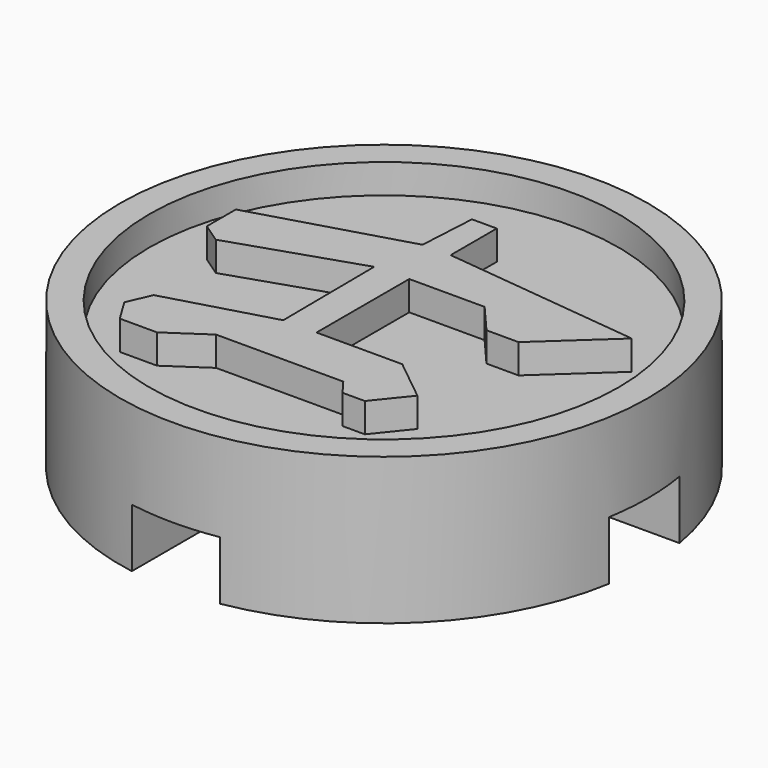
from build123d import *

# Parameters (mm, degrees)
F0_R     = 9
F1_DEPTH = 4
F3_W     = 3
F3_H     = 3
F4_DEPTH = 2
F2_R     = 9
F2_R_2   = 8
F5_DEPTH = 1


with BuildPart() as f1:
    # F0 (on Top) → F1 (new body)
    with BuildSketch(Plane.XY):
        with Locations((-31.3306450844, 19.7580661625)):
            Circle(F0_R)
    extrude(amount=F1_DEPTH)

    # F3 (on face) → F4 (cut)
    with BuildSketch(Plane(origin=(0, 0, 0), x_dir=(1, 0, 0), z_dir=(0, 0, -1))):
        with BuildLine():
            ThreePointArc((-32.8306450844, -28.6321858371), (-32.0832814269, -28.7265408676), (-31.3306450844, -28.7580661625))
            ThreePointArc((-31.3306450844, -28.7580661625), (-30.5780087419, -28.7265408676), (-29.8306450844, -28.6321858371))
            Line((-29.8306450844, -28.6321858371), (-29.8306450844, -21.2580661625))
            Line((-29.8306450844, -21.2580661625), (-32.8306450844, -21.2580661625))
            Line((-32.8306450844, -21.2580661625), (-32.8306450844, -28.6321858371))
        make_face()
        with BuildLine():
            ThreePointArc((-40.204764759, -18.2580661625), (-40.2991197895, -19.0054298199), (-40.3306450844, -19.7580661625))
            ThreePointArc((-40.3306450844, -19.7580661625), (-40.2991197895, -20.510702505), (-40.204764759, -21.2580661625))
            Line((-40.204764759, -21.2580661625), (-32.8306450844, -21.2580661625))
            Line((-32.8306450844, -21.2580661625), (-32.8306450844, -18.2580661625))
            Line((-32.8306450844, -18.2580661625), (-40.204764759, -18.2580661625))
        make_face()
        with Locations((-31.3306450844, -19.7580661625)):
            Rectangle(F3_W, F3_H)
        with BuildLine():
            Line((-29.8306450844, -18.2580661625), (-29.8306450844, -21.2580661625))
            Line((-29.8306450844, -21.2580661625), (-22.4565254097, -21.2580661625))
            ThreePointArc((-22.4565254097, -21.2580661625), (-22.3621703793, -20.510702505), (-22.3306450844, -19.7580661625))
            ThreePointArc((-22.3306450844, -19.7580661625), (-22.3621703793, -19.0054298199), (-22.4565254097, -18.2580661625))
            Line((-22.4565254097, -18.2580661625), (-29.8306450844, -18.2580661625))
        make_face()
        with BuildLine():
            Line((-32.8306450844, -10.8839464878), (-32.8306450844, -18.2580661625))
            Line((-32.8306450844, -18.2580661625), (-29.8306450844, -18.2580661625))
            Line((-29.8306450844, -18.2580661625), (-29.8306450844, -10.8839464878))
            ThreePointArc((-29.8306450844, -10.8839464878), (-30.5780087419, -10.7895914574), (-31.3306450844, -10.7580661625))
            ThreePointArc((-31.3306450844, -10.7580661625), (-32.0832814269, -10.7895914574), (-32.8306450844, -10.8839464878))
        make_face()
    extrude(amount=-F4_DEPTH, mode=Mode.SUBTRACT)

    # F2 (on face) → F5 (join)
    with BuildSketch(Plane.XY.offset(4)):
        with Locations((-31.3306450844, 19.7580661625)):
            Circle(F2_R)
        with Locations((-31.3306450844, 19.7580661625)):
            Circle(F2_R_2, mode=Mode.SUBTRACT)
        Polygon((-31.5887257457, 24.8875524849), (-32.4354991317, 24.8875524849), (-32.5466804206, 22.920306772), (-37.6978889108, 21.4031711221), (-37.6978889108, 20.1682914048), (-37.0275266469, 19.7096224874), (-32.7583737671, 21.1209114641), (-32.7230915427, 17.2045808285), (-36.3218821585, 16.1813963205), (-36.6747044027, 15.3699042276), (-36.1807532609, 14.5584121346), (-34.9105931818, 14.5584121346), (-33.6051471531, 15.4404686764), (-29.2654298246, 15.4404686764), (-28.877325356, 14.9242647582), (-28.1173038363, 14.9242647582), (-27.2190589458, 16.0402674228), (-28.6656320095, 17.2045808285), (-31.5887257457, 17.2045808285), (-31.5887257457, 21.1561955512), (-29.0184542537, 21.1561955512), (-28.1363967806, 20.1330091804), (-27.0426478237, 20.1330091804), (-24.8198658228, 22.1793800592), (-31.5887257457, 22.920306772), align=None)
    extrude(amount=F5_DEPTH)


solid = f1.part
